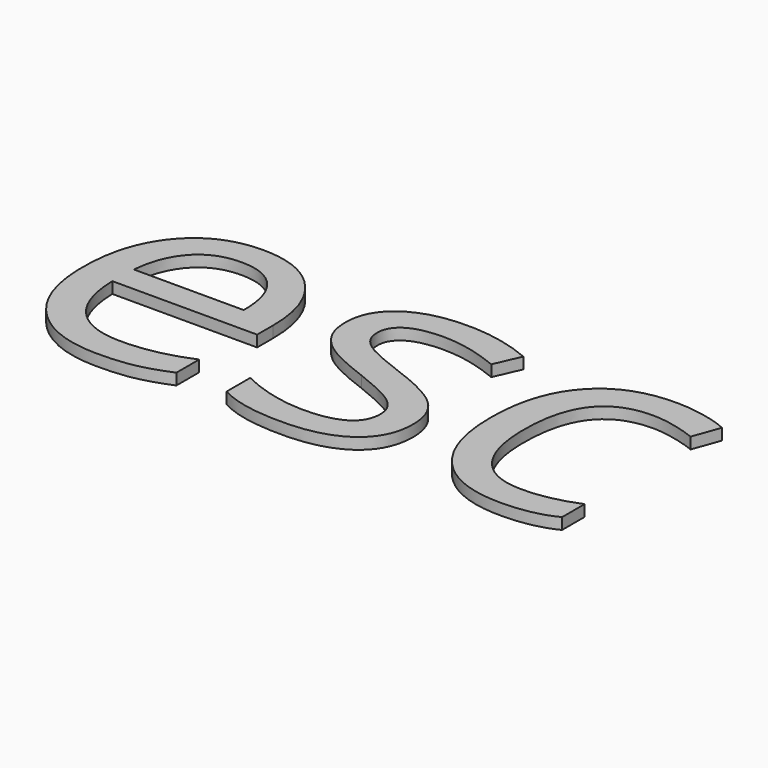
from build123d import *

# Parameters (mm, degrees)
F0_TEXT_SIZE = 8.8194444444
F1_DEPTH     = 0.254


# Not quite as in the source:
# - Text() gives the source's letters only with a copy of the font that has no kerning and outlines rounded to 1/6400 em; it was checked with that copy


with BuildPart() as f1:
    # F0 (on Top) → F1 (new body)
    with BuildSketch(Plane.XY):
        with Locations((-34.0693396779, 12.5883384823)):
            Text('esc', F0_TEXT_SIZE, font='Open Sans', text_align=(TextAlign.LEFT, TextAlign.BOTTOM))
    extrude(amount=F1_DEPTH)


solid = f1.part
